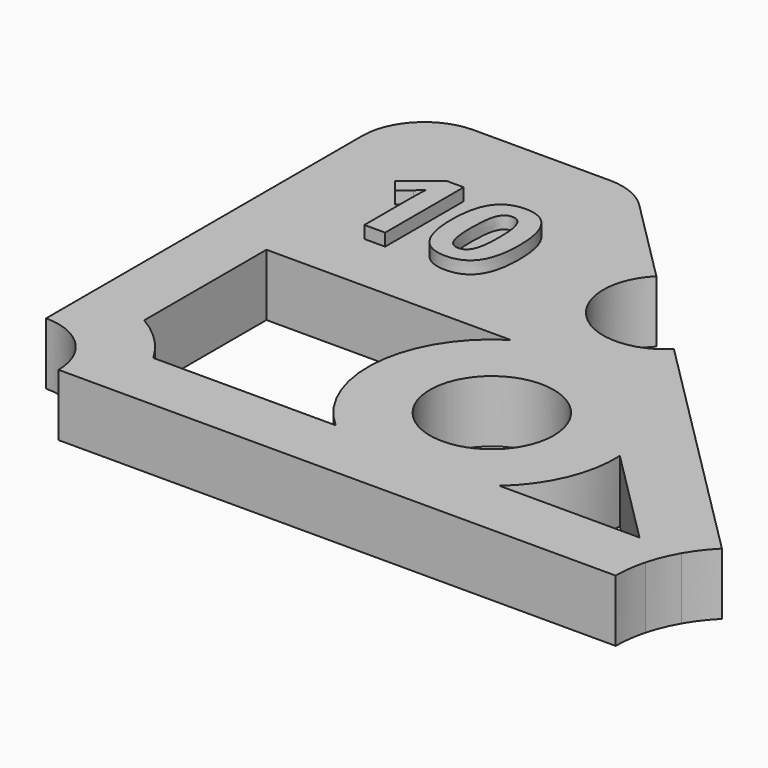
from build123d import *

# Parameters (mm, degrees)
F0_TEXT_SIZE = 11.1111111111
F1_DEPTH     = 5
F2_DEPTH     = 1


# Not quite as in the source:
# - Text() gives the source's letters only with a copy of the font that has no kerning and outlines rounded to 1/6400 em; it was checked with that copy


with BuildPart() as f1:
    # F0 (on Top) → F1 (new body)
    with BuildSketch(Plane.XY):
        with BuildLine():
            ThreePointArc((-25, 11.9289321881), (-28.5355339059, 10.4644660941), (-30, 6.9289321881))
            Line((-30, 6.9289321881), (-30, -20))
            Line((-30, -20), (-30, -25))
            ThreePointArc((-30, -25), (-26.4644660941, -26.4644660941), (-25, -30))
            Line((-25, -30), (-20, -30))
            Line((-20, -30), (20, -30))
            ThreePointArc((20, -30), (20.0855513863, -28.6947380778), (20.3407417371, -27.411809549))
            Line((20.3407417371, -27.411809549), (17.9289321881, -25))
            Line((17.9289321881, -25), (21.3397459622, -25))
            ThreePointArc((21.3397459622, -25), (22.0664665971, -23.9123857099), (22.9289321881, -22.9289321881))
            Line((22.9289321881, -22.9289321881), (3.5355339059, -3.5355339059))
            ThreePointArc((3.5355339059, -3.5355339059), (-3.5355339059, -3.5355339059), (-3.5355339059, 3.5355339059))
            Line((-3.5355339059, 3.5355339059), (-10.4644660941, 10.4644660941))
            ThreePointArc((-10.4644660941, 10.4644660941), (-12.0865828382, 11.5483298507), (-14, 11.9289321881))
            Line((-14, 11.9289321881), (-25, 11.9289321881))
        make_face()
        with BuildLine():
            Line((-5, -9), (-5, -17.5))
            Line((-5, -17.5), (-5, -25))
            Line((-5, -25), (-6.6143782777, -25))
            Line((-6.6143782777, -25), (-21.3397459622, -25))
            ThreePointArc((-21.3397459622, -25), (-22.9289321881, -22.9289321881), (-25, -21.3397459622))
            Line((-25, -21.3397459622), (-25, -9))
            Line((-25, -9), (-5.2678268764, -9))
            Line((-5.2678268764, -9), (-5, -9))
        make_face(mode=Mode.SUBTRACT)
        with BuildLine():
            ThreePointArc((-5, -17.5), (0, -12.5), (5, -17.5))
            ThreePointArc((5, -17.5), (0, -22.5), (-5, -17.5))
        make_face(mode=Mode.SUBTRACT)
        Polygon((9.9903789234, -17.0614467353), (17.9289321881, -25), (6.6143782777, -25), (5, -25), (5, -17.5), (5, -12.0710678119), align=None, mode=Mode.SUBTRACT)
        with BuildLine():
            Line((-19.4140625, 3.9322916667), (-19.4140625, -4))
            Line((-19.4140625, -4), (-21.0911458333, -4))
            Line((-21.0911458333, -4), (-21.0911458333, 0.5902777778))
            Line((-21.0911458333, 0.5902777778), (-21.0737847222, 1.34375))
            Line((-21.0737847222, 1.34375), (-21.0477430556, 2.1684027778))
            add(Edge.make_bspline(
                [(-21.0477430556, 2.1684027778), (-21.4644097222, 1.7517361111), (-21.6276041667, 1.6215277778)],
                knots=[0, 0, 0, 1, 1, 1], degree=2))
            Line((-21.6276041667, 1.6215277778), (-22.5390625, 0.8888888889))
            Line((-22.5390625, 0.8888888889), (-23.3480902778, 1.8975694444))
            Line((-23.3480902778, 1.8975694444), (-20.7925347222, 3.9322916667))
            Line((-20.7925347222, 3.9322916667), (-19.4140625, 3.9322916667))
        make_face(mode=Mode.SUBTRACT)
        with BuildLine():
            add(Edge.make_bspline(
                [(-12.4184027778, 3.015625), (-11.7161458333, 1.9739583333), (-11.7161458333, -0.0347222222)],
                knots=[0, 0, 0, 1, 1, 1], degree=2))
            add(Edge.make_bspline(
                [(-11.7161458333, -0.0347222222), (-11.7161458333, -2.1111111111), (-12.3967013889, -3.1102430556)],
                knots=[0, 0, 0, 1, 1, 1], degree=2))
            add(Edge.make_bspline(
                [(-12.3967013889, -3.1102430556), (-13.0772569444, -4.109375), (-14.4939236111, -4.109375)],
                knots=[0, 0, 0, 1, 1, 1], degree=2))
            add(Edge.make_bspline(
                [(-14.4939236111, -4.109375), (-15.8671875, -4.109375), (-16.5642361111, -3.078125)],
                knots=[0, 0, 0, 1, 1, 1], degree=2))
            add(Edge.make_bspline(
                [(-16.5642361111, -3.078125), (-17.2612847222, -2.046875), (-17.2612847222, -0.0347222222)],
                knots=[0, 0, 0, 1, 1, 1], degree=2))
            add(Edge.make_bspline(
                [(-17.2612847222, -0.0347222222), (-17.2612847222, 2.0659722222), (-16.5824652778, 3.0616319444)],
                knots=[0, 0, 0, 1, 1, 1], degree=2))
            add(Edge.make_bspline(
                [(-16.5824652778, 3.0616319444), (-15.9036458333, 4.0572916667), (-14.4939236111, 4.0572916667)],
                knots=[0, 0, 0, 1, 1, 1], degree=2))
            add(Edge.make_bspline(
                [(-14.4939236111, 4.0572916667), (-13.1206597222, 4.0572916667), (-12.4184027778, 3.015625)],
                knots=[0, 0, 0, 1, 1, 1], degree=2))
        make_face(mode=Mode.SUBTRACT)
        with BuildLine():
            Line((-5, -25), (-5, -17.5))
            Line((-5, -17.5), (-5, -9))
            Line((-5, -9), (-5.2678268764, -9))
            ThreePointArc((-5.2678268764, -9), (-9.9647729443, -16.6613700643), (-6.6143782777, -25))
            Line((-6.6143782777, -25), (-5, -25))
        make_face()
        with BuildLine():
            ThreePointArc((6.6143782777, -25), (9.2024261698, -21.4134834341), (9.9903789234, -17.0614467353))
            Line((9.9903789234, -17.0614467353), (5, -12.0710678119))
            Line((5, -12.0710678119), (5, -17.5))
            Line((5, -17.5), (5, -25))
            Line((5, -25), (6.6143782777, -25))
        make_face()
        with BuildLine():
            Line((17.9289321881, -25), (20.3407417371, -27.411809549))
            ThreePointArc((20.3407417371, -27.411809549), (20.7612046749, -26.1731656763), (21.3397459622, -25))
            Line((21.3397459622, -25), (17.9289321881, -25))
        make_face()
        with Locations((-24.0043402778, -4)):
            Text('10', F0_TEXT_SIZE, font='Open Sans', font_style=FontStyle.BOLD, text_align=(TextAlign.LEFT, TextAlign.BOTTOM))
        with BuildLine():
            add(Edge.make_bspline(
                [(-15.3402777778, 2.0625), (-15.5946180556, 1.4253472222), (-15.5946180556, -0.0347222222)],
                knots=[0, 0, 0, 1, 1, 1], degree=2))
            add(Edge.make_bspline(
                [(-15.5946180556, -0.0347222222), (-15.5946180556, -1.4930555556), (-15.3428819444, -2.125)],
                knots=[0, 0, 0, 1, 1, 1], degree=2))
            add(Edge.make_bspline(
                [(-15.3428819444, -2.125), (-15.0911458333, -2.7569444444), (-14.4939236111, -2.7569444444)],
                knots=[0, 0, 0, 1, 1, 1], degree=2))
            add(Edge.make_bspline(
                [(-14.4939236111, -2.7569444444), (-13.9071180556, -2.7569444444), (-13.6467013889, -2.1171875)],
                knots=[0, 0, 0, 1, 1, 1], degree=2))
            add(Edge.make_bspline(
                [(-13.6467013889, -2.1171875), (-13.3862847222, -1.4774305556), (-13.3862847222, -0.0347222222)],
                knots=[0, 0, 0, 1, 1, 1], degree=2))
            add(Edge.make_bspline(
                [(-13.3862847222, -0.0347222222), (-13.3862847222, 1.4253472222), (-13.6501736111, 2.0625)],
                knots=[0, 0, 0, 1, 1, 1], degree=2))
            add(Edge.make_bspline(
                [(-13.6501736111, 2.0625), (-13.9140625, 2.6996527778), (-14.4939236111, 2.6996527778)],
                knots=[0, 0, 0, 1, 1, 1], degree=2))
            add(Edge.make_bspline(
                [(-14.4939236111, 2.6996527778), (-15.0859375, 2.6996527778), (-15.3402777778, 2.0625)],
                knots=[0, 0, 0, 1, 1, 1], degree=2))
        make_face()
    extrude(amount=-F1_DEPTH)

    # F0 (on Top) → F2 (join)
    with BuildSketch(Plane.XY):
        with Locations((-24.0043402778, -4)):
            Text('10', F0_TEXT_SIZE, font='Open Sans', font_style=FontStyle.BOLD, text_align=(TextAlign.LEFT, TextAlign.BOTTOM))
    extrude(amount=F2_DEPTH)


solid = f1.part
